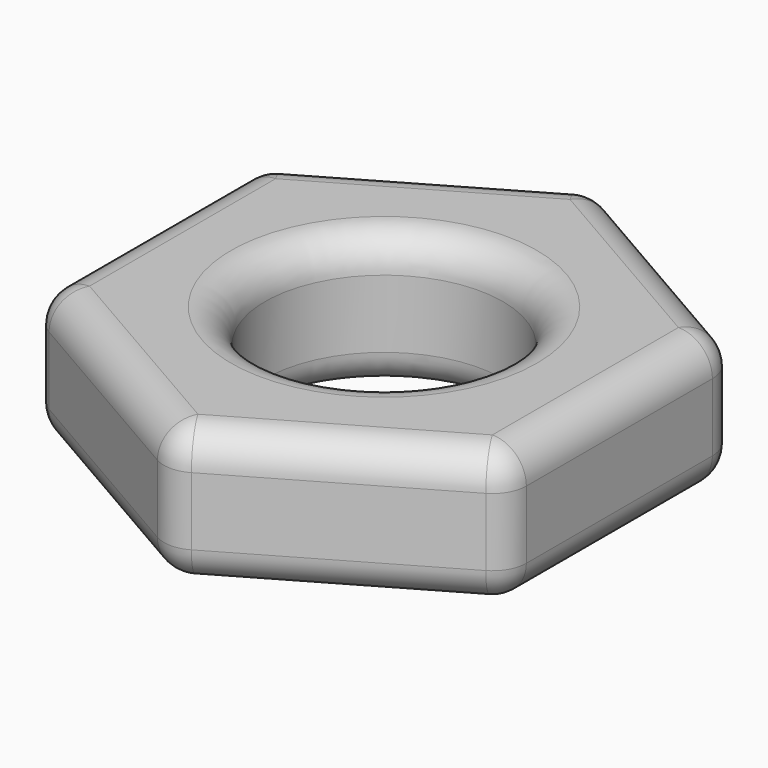
from build123d import *

# Parameters (mm, degrees)
F0_R     = 22.225
F1_DEPTH = 25.4
F2_R     = 6.35
F3_R     = 6.35


# Not quite as in the source:
# - a feature names something its author has since deleted; it is built from what else it names


with BuildPart() as f1:
    # F0 (on Top) → F1 (new body)
    with BuildSketch(Plane.XY):
        Polygon((0, -50.8), (43.9940905122, -25.4), (43.9940905122, 25.4), (0, 50.8), (-43.9940905122, 25.4), (-43.9940905122, -25.4), align=None)
        Circle(F0_R, mode=Mode.SUBTRACT)
    extrude(amount=F1_DEPTH)

    # F2
    f2_edges = [f1.edges().sort_by_distance(p)[0] for p in [
        (-43.994091, -25.4, 12.7),
        (-43.994091, 25.4, 12.7),
        (0, -50.8, 12.7),
        (43.994091, -25.4, 12.7),
        (43.994091, 25.4, 12.7),
        (0, 50.8, 12.7),
    ]]
    fillet(f2_edges, radius=F2_R)

    # F3
    f3_edges = [f1.edges().sort_by_distance(p)[0] for p in [
        (-21.997045, -38.1, 25.4),
        (-21.997045, -38.1, 0),
        (-22.225, 0, 25.4),
        (-22.225, 0, 0),
    ]]
    fillet(f3_edges, radius=F3_R)


solid = f1.part
